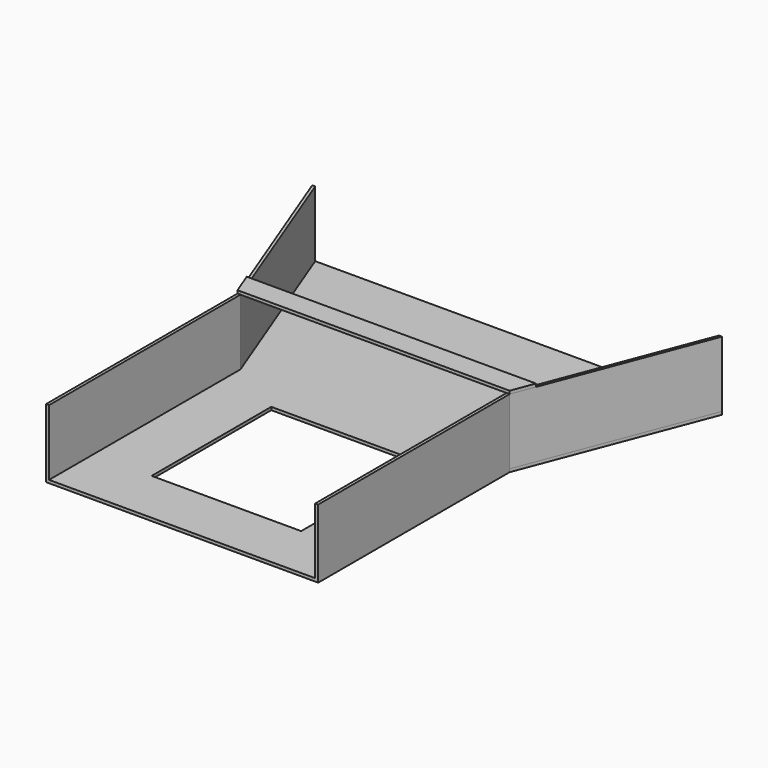
from build123d import *

# Parameters (mm, degrees)
F0_W      = 288.925
F0_H      = 190.5
F1_DEPTH  = 3.175
F3_DEPTH  = 3.175
F5_DEPTH  = 3.175
F6_W      = 288.925
F6_H      = 254
F7_DEPTH  = 3.175
F8_W      = 158.75
F8_H      = 158.75
F9_DEPTH  = 3.175
F12_DEPTH = 69.85
F13_W     = 3.1750007891
F13_H     = 253.9999979416
F13_W_2   = 3.1750009115
F13_H_2   = 253.9999979885
F14_DEPTH = 69.85
F16_DEPTH = 3.175


# Not quite as in the source:
# - ends of sketch curves that miss each other by under 0.0002 mm in the source are joined


with BuildPart() as f1:
    # F0 (on Top) → F1 (new body)
    with BuildSketch(Plane.XY):
        Rectangle(F0_W, F0_H)
    extrude(amount=F1_DEPTH)

    # F2 (on face) → F3 (join)
    with BuildSketch(Plane.XY.offset(3.175)):
        Polygon((-144.4625, -95.25), (-144.4625, 95.25), (-217.4875, 95.25), align=None)
    extrude(amount=-F3_DEPTH)

    # F4 (on face) → F5 (join)
    with BuildSketch(Plane(origin=(0, 0, 0), x_dir=(1, 0, 0), z_dir=(0, 0, -1))):
        Polygon((217.4875, -95.25), (144.4625, 95.25), (144.4625, -95.25), align=None)
    extrude(amount=-F5_DEPTH)

    # F6 (on face) → F7 (join)
    with BuildSketch(Plane.XY.offset(3.175)):
        with Locations((0, -222.25)):
            Rectangle(F6_W, F6_H)
    extrude(amount=-F7_DEPTH)

    # F8 (on face) → F9 (cut)
    with BuildSketch(Plane.XY.offset(3.175)):
        with Locations((0, -211.1248)):
            Rectangle(F8_W, F8_H)
    extrude(amount=-F9_DEPTH, mode=Mode.SUBTRACT)

    # F10 (on face) + F11 (on face) → F12 (join)
    with BuildSketch(Plane.XY.offset(3.175)):
        Polygon((-214.3125, 95.25), (-217.4875, 95.25), (-144.4624992109, -95.2500020584), (-141.2874992109, -95.2500020584), align=None)
    with BuildSketch(Plane.XY.offset(3.175)):
        Polygon((144.4624990885, -95.2500020115), (217.4875, 95.25), (214.3125, 95.25), (141.2874990885, -95.2500020115), align=None)
    extrude(amount=F12_DEPTH)

    # F13 (on face) → F14 (join)
    with BuildSketch(Plane.XY.offset(3.175)):
        with Locations((-142.8749996055, -222.2500010292)):
            Rectangle(F13_W, F13_H)
        with Locations((142.8749995443, -222.2500010058)):
            Rectangle(F13_W_2, F13_H_2)
    extrude(amount=F14_DEPTH)

    # F15 (on face) → F16 (join)
    with BuildSketch(Plane.XY.offset(73.025)):
        Polygon((-153.5540740075, -71.5328504152), (-144.4625, -95.25), (-141.2874992109, -95.2500000226), (-150.3790740075, -71.5328504152), align=None)
        Polygon((-150.3790740075, -71.5328504152), (-141.2874992109, -95.2500020584), (144.4625, -95.2500020584), (153.5540740075, -71.5328504152), align=None)
    extrude(amount=F16_DEPTH)


solid = f1.part
